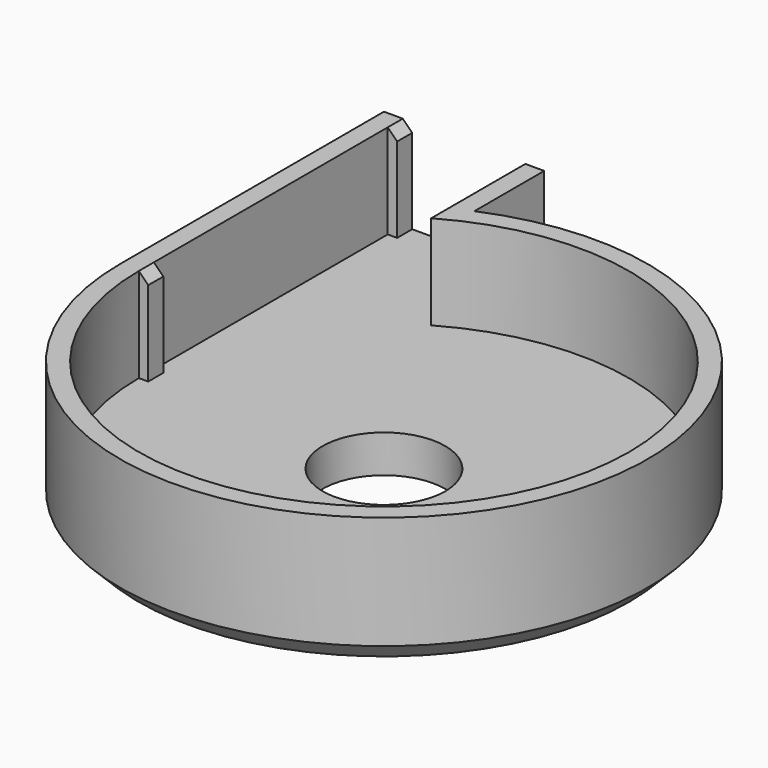
from build123d import *

# Parameters (mm, degrees)
F0_R      = 14
F0_R_2    = 3.25
F1_DEPTH  = 7
F2_R      = 13
F3_DEPTH  = 5
F5_DEPTH  = 7
F6_W      = 8.5
F6_H      = 2
F7_DEPTH  = 12.8
F8_W      = 6.5
F8_H      = 5
F9_DEPTH  = 17.5
F10_W     = 1
F10_H     = 5
F11_DEPTH = 0.5
F12_W     = 1
F12_H     = 5
F13_DEPTH = 0.5
F14_SIZE  = 0.49999
F15_SIZE  = 1


# Not quite as in the source:
# - a fillet or chamfer is up to 0.001 mm smaller than in the source, because OpenCascade refuses the exact size


with BuildPart() as f1:
    # F0 (on Top) → F1 (new body)
    with BuildSketch(Plane.XY):
        Circle(F0_R)
        Circle(F0_R_2, mode=Mode.SUBTRACT)
    extrude(amount=F1_DEPTH)

    # F2 (on face) → F3 (cut)
    with BuildSketch(Plane.XY.offset(7)):
        Circle(F2_R)
    extrude(amount=-F3_DEPTH, mode=Mode.SUBTRACT)

    # F4 (on face) → F5 (join)
    with BuildSketch(Plane.XY.offset(7)):
        with BuildLine():
            Line((-14, 17.5), (-14, 0))
            ThreePointArc((-14, 0), (-13.7477270849, 2.6457513111), (-13, 5.1961524227))
            Line((-13, 5.1961524227), (-13, 17.5))
            Line((-13, 17.5), (-14, 17.5))
        make_face()
        with BuildLine():
            ThreePointArc((-6.5, 12.3995967676), (-6.0046946559, 12.6468827024), (-5.5, 12.8743931896))
            Line((-5.5, 12.8743931896), (-5.5, 17.5))
            Line((-5.5, 17.5), (-6.5, 17.5))
            Line((-6.5, 17.5), (-6.5, 12.3995967676))
        make_face()
    extrude(amount=-F5_DEPTH)

    # F6 (on face) → F7 (join)
    with BuildSketch(Plane(origin=(0, 17.5, 0), x_dir=(-1, 0, 0), z_dir=(0, 1, 0))):
        with Locations((9.75, 1)):
            Rectangle(F6_W, F6_H)
    extrude(amount=-F7_DEPTH)

    # F8 (on face) → F9 (cut)
    with BuildSketch(Plane(origin=(0, 17.5, 0), x_dir=(-1, 0, 0), z_dir=(0, 1, 0))):
        with Locations((9.75, 4.5)):
            Rectangle(F8_W, F8_H)
    extrude(amount=-F9_DEPTH, mode=Mode.SUBTRACT)

    # F10 (on face) → F11 (join)
    with BuildSketch(Plane.YZ.offset(-13)):
        with Locations((0.5, 4.5)):
            Rectangle(F10_W, F10_H)
        with Locations((17, 4.5)):
            Rectangle(F10_W, F10_H)
    extrude(amount=F11_DEPTH)

    # F12 (on face) → F13 (join)
    with BuildSketch(Plane(origin=(-6.5, 0, 0), x_dir=(0, -1, 0), z_dir=(-1, 0, 0))):
        with Locations((-17, 4.5)):
            Rectangle(F12_W, F12_H)
    extrude(amount=F13_DEPTH)

    # F14 (size 0.5 in the source; OpenCascade refuses exactly that, so slightly less here)
    f14_edges = [f1.edges().sort_by_distance(p)[0] for p in [
        (-12.5, 0.5, 7),
        (-12.5, 17, 7),
        (-7, 17, 7),
    ]]
    chamfer(f14_edges, length=F14_SIZE)

    # F15
    f15_edges = [f1.edges().sort_by_distance(p)[0] for p in [
        (11.683321, -7.713624, 0),
        (-5.5, 15.187197, 0),
        (-14, 8.75, 0),
    ]]
    chamfer(f15_edges, length=F15_SIZE)


solid = f1.part
